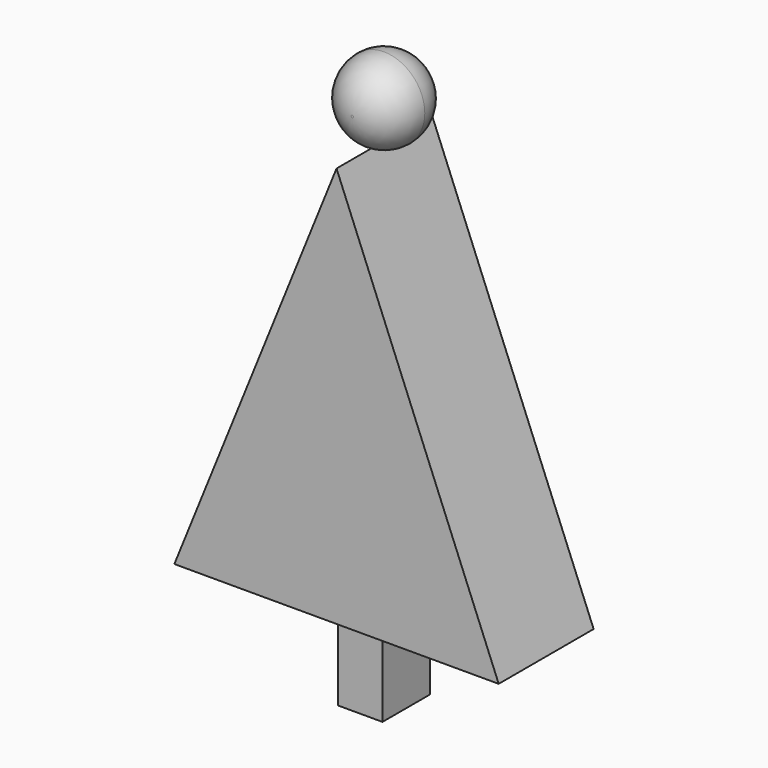
from build123d import *

# Parameters (mm, degrees)
F0_R     = 5.2363216072
F3_DEPTH = 5.08
F4_R     = 5.07999
F2_W     = 5.7048136368
F2_H     = 11.6948671639
F6_DEPTH = 3.81
F7_DEPTH = 7.62


# Not quite as in the source:
# - a fillet or chamfer is up to 0.001 mm smaller than in the source, because OpenCascade refuses the exact size


with BuildPart() as f3:
    # F0 (on Front) → F3 (new body)
    with BuildSketch(Plane.XZ):
        with Locations((0, 56.3350282609)):
            Circle(F0_R)
    extrude(amount=F3_DEPTH)

    # F4 (radius 5.08 in the source; OpenCascade refuses exactly that, so slightly less here)
    f4_edges = [f3.edges().sort_by_distance(p)[0] for p in [
        (-5.236322, -5.08, 56.335028),
    ]]
    fillet(f4_edges, radius=F4_R)

    # F5: F3 across plane


with BuildPart() as f3_1:
    add(f3.part)
    add(f3.part.mirror(Plane.XZ))


with BuildPart() as f6:
    # F2 (on Front) → F6 (new body, symmetric)
    with BuildSketch(Plane.XZ):
        with Locations((0, -5.8474335819)):
            Rectangle(F2_W, F2_H)
    extrude(amount=F6_DEPTH, both=True)


with BuildPart() as f7:
    # F1 (on Front) → F7 (new body, symmetric)
    with BuildSketch(Plane.XZ):
        Polygon((20.8225678653, 0), (0, 51.4859370887), (-20.8225660026, 0), align=None)
    extrude(amount=F7_DEPTH, both=True)


solid = Compound([f3_1.part, f6.part, f7.part])
